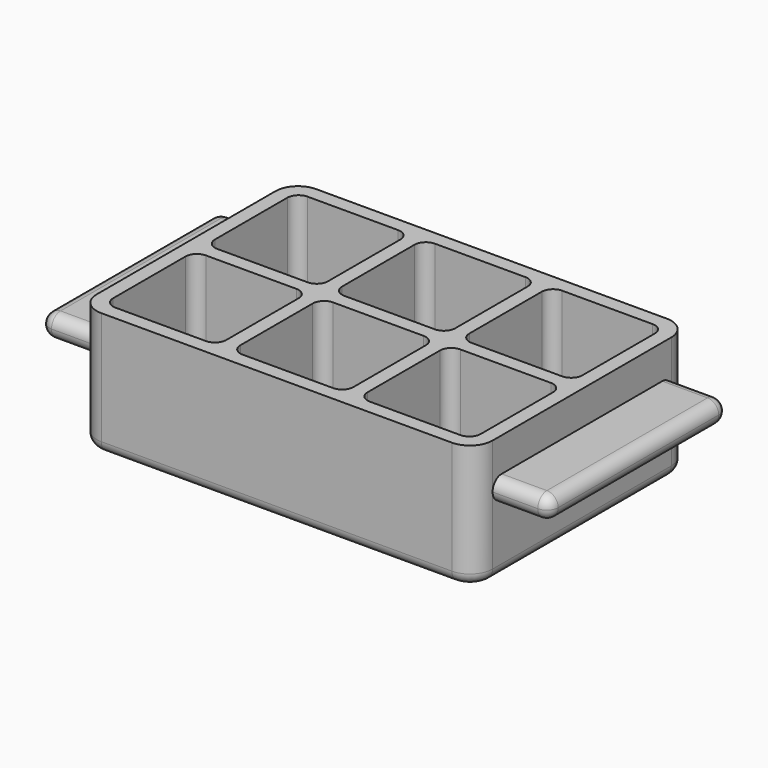
from build123d import *

# Parameters (mm, degrees)
F0_W     = 50.8
F0_H     = 50.8
F1_DEPTH = 5.08
F0_W_2   = 177.8
F0_H_2   = 120.65
F2_DEPTH = 55.88
F3_R     = 10.16
F4_R     = 5.08
F5_W     = 100.33
F5_H     = 10.16
F6_DEPTH = 25.4
F7_R     = 5.07999
F8_W     = 100.33
F8_H     = 10.16
F9_DEPTH = 25.4
F10_R    = 5.07999


# Not quite as in the source:
# - a fillet or chamfer is up to 0.001 mm smaller than in the source, because OpenCascade refuses the exact size


with BuildPart() as f1:
    # F0 (on Top) → F1 (new body)
    with BuildSketch(Plane.XY):
        with Locations((71.5988487065, -31.75)):
            Rectangle(F0_W, F0_H)
    extrude(amount=F1_DEPTH)


with BuildPart() as f1b:
    # F0 (on Top) → F1, piece 2 (new body)
    with BuildSketch(Plane.XY):
        with Locations((14.4488487065, -31.75)):
            Rectangle(F0_W, F0_H)
    extrude(amount=F1_DEPTH)


with BuildPart() as f1c:
    # F0 (on Top) → F1, piece 3 (new body)
    with BuildSketch(Plane.XY):
        with Locations((-42.7011512935, -31.75)):
            Rectangle(F0_W, F0_H)
    extrude(amount=F1_DEPTH)


with BuildPart() as f1d:
    # F0 (on Top) → F1, piece 4 (new body)
    with BuildSketch(Plane.XY):
        with Locations((-42.7011512935, 25.4)):
            Rectangle(F0_W, F0_H)
    extrude(amount=F1_DEPTH)


with BuildPart() as f1e:
    # F0 (on Top) → F1, piece 5 (new body)
    with BuildSketch(Plane.XY):
        with Locations((14.4488487065, 25.4)):
            Rectangle(F0_W, F0_H)
    extrude(amount=F1_DEPTH)


with BuildPart() as f1f:
    # F0 (on Top) → F1, piece 6 (new body)
    with BuildSketch(Plane.XY):
        with Locations((71.5988487065, 25.4)):
            Rectangle(F0_W, F0_H)
    extrude(amount=F1_DEPTH)


with BuildPart() as f2:
    # F0 (on Top) → F2 (new body)
    with BuildSketch(Plane.XY):
        with Locations((14.4488487065, -3.175)):
            Rectangle(F0_W_2, F0_H_2)
        with Locations((-42.7011512935, -31.75)):
            Rectangle(F0_W, F0_H, mode=Mode.SUBTRACT)
        with Locations((14.4488487065, -31.75)):
            Rectangle(F0_W, F0_H, mode=Mode.SUBTRACT)
        with Locations((71.5988487065, -31.75)):
            Rectangle(F0_W, F0_H, mode=Mode.SUBTRACT)
        with Locations((-42.7011512935, 25.4)):
            Rectangle(F0_W, F0_H, mode=Mode.SUBTRACT)
        with Locations((14.4488487065, 25.4)):
            Rectangle(F0_W, F0_H, mode=Mode.SUBTRACT)
        with Locations((71.5988487065, 25.4)):
            Rectangle(F0_W, F0_H, mode=Mode.SUBTRACT)
    extrude(amount=F2_DEPTH)

    # F3
    f3_edges = [f2.edges().sort_by_distance(p)[0] for p in [
        (103.348849, -63.5, 27.94),
        (103.348849, 57.15, 27.94),
        (-74.451151, 57.15, 27.94),
        (-74.451151, -63.5, 27.94),
    ]]
    fillet(f3_edges, radius=F3_R)

    # F4 (call 1 of 25: OpenCascade refuses the feature's edges together)
    f4_edges = [f2.edges().sort_by_distance(p)[0] for p in [
        (-17.301151, -6.35, 27.94),
    ]]
    fillet(f4_edges, radius=F4_R)

    # F4#2 (call 2 of 25)
    f4_2_edges = [f2.edges().sort_by_distance(p)[0] for p in [
        (-17.301151, 50.8, 27.94),
    ]]
    fillet(f4_2_edges, radius=F4_R)

    # F4#3 (call 3 of 25)
    f4_3_edges = [f2.edges().sort_by_distance(p)[0] for p in [
        (39.848849, 50.8, 27.94),
    ]]
    fillet(f4_3_edges, radius=F4_R)

    # F4#4 (call 4 of 25)
    f4_4_edges = [f2.edges().sort_by_distance(p)[0] for p in [
        (96.998849, 50.8, 27.94),
    ]]
    fillet(f4_4_edges, radius=F4_R)

    # F4#5 (call 5 of 25)
    f4_5_edges = [f2.edges().sort_by_distance(p)[0] for p in [
        (96.998849, -6.35, 27.94),
    ]]
    fillet(f4_5_edges, radius=F4_R)

    # F4#6 (call 6 of 25)
    f4_6_edges = [f2.edges().sort_by_distance(p)[0] for p in [
        (39.848849, -6.35, 27.94),
    ]]
    fillet(f4_6_edges, radius=F4_R)

    # F4#7 (call 7 of 25)
    f4_7_edges = [f2.edges().sort_by_distance(p)[0] for p in [
        (96.998849, 0, 27.94),
    ]]
    fillet(f4_7_edges, radius=F4_R)

    # F4#8 (call 8 of 25)
    f4_8_edges = [f2.edges().sort_by_distance(p)[0] for p in [
        (39.848849, 0, 27.94),
    ]]
    fillet(f4_8_edges, radius=F4_R)

    # F4#9 (call 9 of 25)
    f4_9_edges = [f2.edges().sort_by_distance(p)[0] for p in [
        (-17.301151, 0, 27.94),
    ]]
    fillet(f4_9_edges, radius=F4_R)

    # F4#10 (call 10 of 25)
    f4_10_edges = [f2.edges().sort_by_distance(p)[0] for p in [
        (-17.301151, -57.15, 27.94),
    ]]
    fillet(f4_10_edges, radius=F4_R)

    # F4#11 (call 11 of 25)
    f4_11_edges = [f2.edges().sort_by_distance(p)[0] for p in [
        (39.848849, -57.15, 27.94),
    ]]
    fillet(f4_11_edges, radius=F4_R)

    # F4#12 (call 12 of 25)
    f4_12_edges = [f2.edges().sort_by_distance(p)[0] for p in [
        (96.998849, -57.15, 27.94),
    ]]
    fillet(f4_12_edges, radius=F4_R)

    # F4#13 (call 13 of 25)
    f4_13_edges = [f2.edges().sort_by_distance(p)[0] for p in [
        (46.198849, -57.15, 27.94),
    ]]
    fillet(f4_13_edges, radius=F4_R)

    # F4#14 (call 14 of 25)
    f4_14_edges = [f2.edges().sort_by_distance(p)[0] for p in [
        (46.198849, 0, 27.94),
    ]]
    fillet(f4_14_edges, radius=F4_R)

    # F4#15 (call 15 of 25)
    f4_15_edges = [f2.edges().sort_by_distance(p)[0] for p in [
        (-10.951151, -57.15, 27.94),
    ]]
    fillet(f4_15_edges, radius=F4_R)

    # F4#16 (call 16 of 25)
    f4_16_edges = [f2.edges().sort_by_distance(p)[0] for p in [
        (-10.951151, 0, 27.94),
    ]]
    fillet(f4_16_edges, radius=F4_R)

    # F4#17 (call 17 of 25)
    f4_17_edges = [f2.edges().sort_by_distance(p)[0] for p in [
        (-68.101151, 0, 27.94),
    ]]
    fillet(f4_17_edges, radius=F4_R)

    # F4#18 (call 18 of 25)
    f4_18_edges = [f2.edges().sort_by_distance(p)[0] for p in [
        (-68.101151, -57.15, 27.94),
    ]]
    fillet(f4_18_edges, radius=F4_R)

    # F4#19 (call 19 of 25)
    f4_19_edges = [f2.edges().sort_by_distance(p)[0] for p in [
        (46.198849, -6.35, 27.94),
    ]]
    fillet(f4_19_edges, radius=F4_R)

    # F4#20 (call 20 of 25)
    f4_20_edges = [f2.edges().sort_by_distance(p)[0] for p in [
        (46.198849, 50.8, 27.94),
    ]]
    fillet(f4_20_edges, radius=F4_R)

    # F4#21 (call 21 of 25)
    f4_21_edges = [f2.edges().sort_by_distance(p)[0] for p in [
        (-10.951151, 50.8, 27.94),
    ]]
    fillet(f4_21_edges, radius=F4_R)

    # F4#22 (call 22 of 25)
    f4_22_edges = [f2.edges().sort_by_distance(p)[0] for p in [
        (-10.951151, -6.35, 27.94),
    ]]
    fillet(f4_22_edges, radius=F4_R)

    # F4#23 (call 23 of 25)
    f4_23_edges = [f2.edges().sort_by_distance(p)[0] for p in [
        (-68.101151, -6.35, 27.94),
    ]]
    fillet(f4_23_edges, radius=F4_R)

    # F4#24 (call 24 of 25)
    f4_24_edges = [f2.edges().sort_by_distance(p)[0] for p in [
        (-68.101151, 50.8, 27.94),
    ]]
    fillet(f4_24_edges, radius=F4_R)

    # F4#25 (call 25 of 25)
    f4_25_edges = [f2.edges().sort_by_distance(p)[0] for p in [
        (103.348849, -3.175, 0),
        (14.448849, -63.5, 0),
    ]]
    fillet(f4_25_edges, radius=F4_R)

    # F5 (on face) → F6 (join)
    with BuildSketch(Plane.YZ.offset(103.3488487065)):
        with Locations((-3.175, 35.56)):
            Rectangle(F5_W, F5_H)
    extrude(amount=F6_DEPTH)

    # F7 (radius 5.08 in the source; OpenCascade refuses exactly that, so slightly less here)
    f7_edges = [f2.edges().sort_by_distance(p)[0] for p in [
        (128.748849, -3.175, 40.64),
        (116.048849, -53.34, 40.64),
        (128.748849, -53.34, 35.56),
        (116.048849, -53.34, 30.48),
        (128.748849, -3.175, 30.48),
        (116.048849, 46.99, 40.64),
        (116.048849, 46.99, 30.48),
        (128.748849, 46.99, 35.56),
    ]]
    fillet(f7_edges, radius=F7_R)

    # F8 (on face) → F9 (join)
    with BuildSketch(Plane(origin=(-74.4511512935, 0, 0), x_dir=(0, -1, 0), z_dir=(-1, 0, 0))):
        with Locations((3.175, 35.56)):
            Rectangle(F8_W, F8_H)
    extrude(amount=F9_DEPTH)

    # F10 (radius 5.08 in the source; OpenCascade refuses exactly that, so slightly less here)
    f10_edges = [f2.edges().sort_by_distance(p)[0] for p in [
        (-99.851151, -3.175, 40.64),
        (-99.851151, -3.175, 30.48),
        (-99.851151, -53.34, 35.56),
        (-87.151151, -53.34, 40.64),
        (-87.151151, -53.34, 30.48),
        (-87.151151, 46.99, 30.48),
        (-87.151151, 46.99, 40.64),
        (-99.851151, 46.99, 35.56),
    ]]
    fillet(f10_edges, radius=F10_R)


solid = Compound([f1.part, f1b.part, f1c.part, f1d.part, f1e.part, f1f.part, f2.part])
